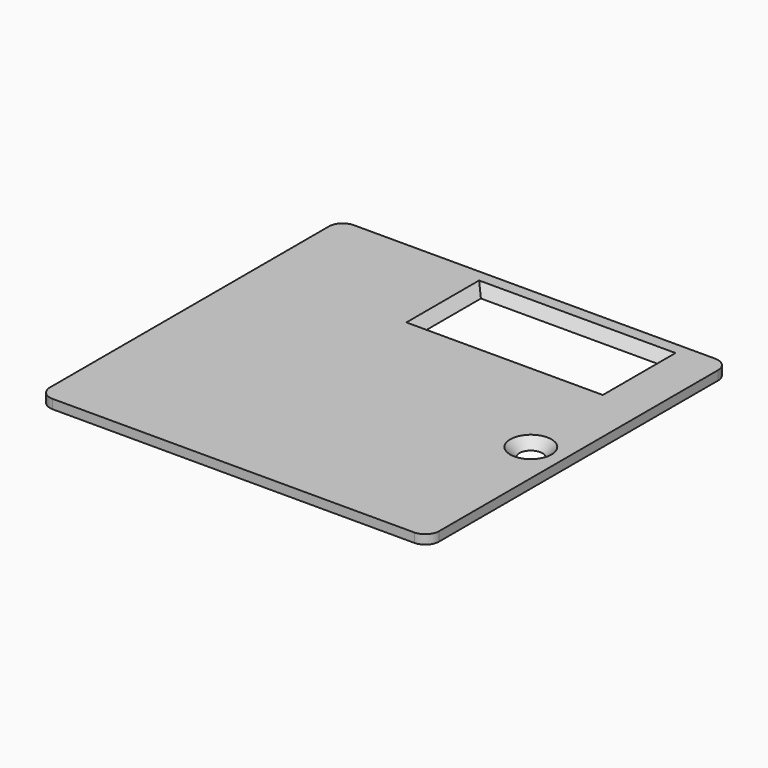
from build123d import *

# Parameters (mm, degrees)
F1_DEPTH     = 2
F2_R         = 3
F0_W         = 55
F0_H         = 20
F0_W_2       = 38
F0_H_2       = 15
F3_DEPTH     = 2
F4_R         = 3
F5_T1_DEPTH  = 38
F5_T3_DEPTH  = 15
F5_T9_DEPTH  = 44.1720391711
F5_T13_DEPTH = 21.1720391711
F5_T20_DEPTH = 44.1720391711
F5_T24_DEPTH = 21.1720391711
F5_T31_DEPTH = 21.1720391711
F5_T35_DEPTH = 44.1720391711
F5_T42_DEPTH = 44.1720391711
F5_T46_DEPTH = 21.1720391711
F8_START     = -23.1
F7_W         = 7.2
F7_H         = 3.4
F8_DEPTH     = 9.4
F9_START     = -23.1
F7_H_2       = 2.4
F9_DEPTH     = 11.8
F10_SIZE     = 2
F11_T4_DEPTH = 17.4867319519
F11_T9_DEPTH = 17.4867319519


# Not quite as in the source:
# - a fillet or chamfer that OpenCascade refuses, or shapes differently, is made with other operations: its cross-section is extruded or revolved along the edge and cut away or added
# - a feature names something its author has since deleted; it is built from what else it names


with BuildPart() as f1:
    # F0 (on Top) → F1 (new body)
    with BuildSketch(Plane.XY):
        with BuildLine():
            Line((42.8, 7.5), (46.1, 7.5))
            Line((46.1, 7.5), (46.1, 21.5))
            Line((46.1, 21.5), (-8.9, 21.5))
            Line((-8.9, 21.5), (-8.9, 41.5))
            Line((-8.9, 41.5), (-30.9, 41.5))
            Line((-30.9, 41.5), (-30.9, -33.5))
            Line((-30.9, -33.5), (46.1, -33.5))
            Line((46.1, -33.5), (46.1, -7.5))
            Line((46.1, -7.5), (42.8, -7.5))
            ThreePointArc((42.8, -7.5), (35.3, 0), (42.8, 7.5))
        make_face()
    extrude(amount=-F1_DEPTH)

    # F2
    f2_edges = [f1.edges().sort_by_distance(p)[0] for p in [
        (46.1, -33.5, -1),
        (-30.9, -33.5, -1),
        (-30.9, 41.5, -1),
    ]]
    fillet(f2_edges, radius=F2_R)

    # F0 (on Top) → F3 (join)
    with BuildSketch(Plane.XY):
        with Locations((18.6, 31.5)):
            Rectangle(F0_W, F0_H)
        with Locations((19, 32.5)):
            Rectangle(F0_W_2, F0_H_2, mode=Mode.SUBTRACT)
        with BuildLine():
            Line((42.8, 7.5), (46.1, 7.5))
            Line((46.1, 7.5), (46.1, 21.5))
            Line((46.1, 21.5), (-8.9, 21.5))
            Line((-8.9, 21.5), (-8.9, 41.5))
            Line((-8.9, 41.5), (-30.9, 41.5))
            Line((-30.9, 41.5), (-30.9, -33.5))
            Line((-30.9, -33.5), (46.1, -33.5))
            Line((46.1, -33.5), (46.1, -7.5))
            Line((46.1, -7.5), (42.8, -7.5))
            ThreePointArc((42.8, -7.5), (35.3, 0), (42.8, 7.5))
        make_face()
        with BuildLine():
            Line((42.8, 1.5), (42.8, 7.5))
            ThreePointArc((42.8, 7.5), (35.3, 0), (42.8, -7.5))
            Line((42.8, -7.5), (42.8, -1.5))
            ThreePointArc((42.8, -1.5), (41.3, 0), (42.8, 1.5))
        make_face()
        with BuildLine():
            Line((46.1, -6.7349832962), (46.1, 6.7349832962))
            ThreePointArc((46.1, 6.7349832962), (44.4937569599, 7.3062430401), (42.8, 7.5))
            Line((42.8, 7.5), (42.8, 1.5))
            ThreePointArc((42.8, 1.5), (43.8606601718, 1.0606601718), (44.3, 0))
            ThreePointArc((44.3, 0), (43.8606601718, -1.0606601718), (42.8, -1.5))
            Line((42.8, -1.5), (42.8, -7.5))
            ThreePointArc((42.8, -7.5), (44.4937569599, -7.3062430401), (46.1, -6.7349832962))
        make_face()
        with BuildLine():
            Line((46.1, -7.5), (46.1, -6.7349832962))
            ThreePointArc((46.1, -6.7349832962), (44.4937569599, -7.3062430401), (42.8, -7.5))
            Line((42.8, -7.5), (46.1, -7.5))
        make_face()
        with BuildLine():
            Line((50, 45), (-34.8, 45))
            Line((-34.8, 45), (-34.8, -37))
            Line((-34.8, -37), (50, -37))
            Line((50, -37), (50, -2.1))
            ThreePointArc((50, -2.1), (48.538751392, -4.8287402561), (46.1, -6.7349832962))
            Line((46.1, -6.7349832962), (46.1, -7.5))
            Line((46.1, -7.5), (46.1, -33.5))
            Line((46.1, -33.5), (-30.9, -33.5))
            Line((-30.9, -33.5), (-30.9, 41.5))
            Line((-30.9, 41.5), (-8.9, 41.5))
            Line((-8.9, 41.5), (46.1, 41.5))
            Line((46.1, 41.5), (46.1, 21.5))
            Line((46.1, 21.5), (46.1, 7.5))
            Line((46.1, 7.5), (46.1, 6.7349832962))
            ThreePointArc((46.1, 6.7349832962), (48.538751392, 4.8287402561), (50, 2.1))
            Line((50, 2.1), (50, 45))
        make_face()
        with BuildLine():
            Line((50, -2.1), (50, 2.1))
            ThreePointArc((50, 2.1), (48.538751392, 4.8287402561), (46.1, 6.7349832962))
            Line((46.1, 6.7349832962), (46.1, -6.7349832962))
            ThreePointArc((46.1, -6.7349832962), (48.538751392, -4.8287402561), (50, -2.1))
        make_face()
        with BuildLine():
            ThreePointArc((42.8, 7.5), (44.4937569599, 7.3062430401), (46.1, 6.7349832962))
            Line((46.1, 6.7349832962), (46.1, 7.5))
            Line((46.1, 7.5), (42.8, 7.5))
        make_face()
    extrude(amount=F3_DEPTH)

    # F4
    f4_edges = [f1.edges().sort_by_distance(p)[0] for p in [
        (50, -37, 1),
        (-34.8, -37, 1),
        (-34.8, 45, 1),
        (50, 45, 1),
    ]]
    fillet(f4_edges, radius=F4_R)

    # F5: chamfer of 2.4 on 4 edges, made by hand

    # F5_s2 → F5_t1 (cut)
    with BuildSketch(Plane.YZ):
        Polygon((42.4, 2), (40, -0.4), (40, 2), align=None)
        Polygon((22.6, 2), (25, -0.4), (25, 2), align=None)
    extrude(amount=F5_T1_DEPTH, mode=Mode.SUBTRACT)

    # F5_s4 → F5_t3 (cut)
    with BuildSketch(Plane.XZ.offset(-40)):
        Polygon((40.4, 2), (38, -0.4), (38, 2), align=None)
        Polygon((-2.4, 2), (0, -0.4), (0, 2), align=None)
    extrude(amount=F5_T3_DEPTH, mode=Mode.SUBTRACT)


with BuildPart() as f5_tool7:
    # F5_s8 → F5_t9 (new body)
    with BuildSketch(Plane.YZ.offset(-6.1720391711)):
        Polygon((42.4, 2), (40, -0.4), (40, 2), align=None)
    extrude(amount=F5_T9_DEPTH)

    split(bisect_by=Plane.YZ, keep=Keep.BOTTOM)


with BuildPart() as f5_tool11:
    # F5_s12 → F5_t13 (new body)
    with BuildSketch(Plane.XZ.offset(-25)):
        Polygon((-2.4, 2), (0, -0.4), (0, 2), align=None)
    extrude(amount=-F5_T13_DEPTH)

    split(bisect_by=Plane.XZ.offset(-40), keep=Keep.BOTTOM)


with BuildPart() as f5_tool7_1:
    add(f5_tool7.part)

    # F5_t15: intersect F5_tool11
    add(f5_tool11.part, mode=Mode.INTERSECT)


with BuildPart() as f1_1:
    add(f1.part)

    # F5_t5: cut F5_tool7
    add(f5_tool7_1.part, mode=Mode.SUBTRACT)


with BuildPart() as f5_tool18:
    # F5_s19 → F5_t20 (new body)
    with BuildSketch(Plane.YZ):
        Polygon((42.4, 2), (40, -0.4), (40, 2), align=None)
    extrude(amount=F5_T20_DEPTH)

    split(bisect_by=Plane.YZ.offset(38), keep=Keep.TOP)


with BuildPart() as f5_tool22:
    # F5_s23 → F5_t24 (new body)
    with BuildSketch(Plane.XZ.offset(-46.1720391711)):
        Polygon((40.4, 2), (38, -0.4), (38, 2), align=None)
    extrude(amount=F5_T24_DEPTH)

    split(bisect_by=Plane.XZ.offset(-40), keep=Keep.BOTTOM)


with BuildPart() as f5_tool18_1:
    add(f5_tool18.part)

    # F5_t26: intersect F5_tool22
    add(f5_tool22.part, mode=Mode.INTERSECT)


with BuildPart() as f1_2:
    add(f1_1.part)

    # F5_t16: cut F5_tool18
    add(f5_tool18_1.part, mode=Mode.SUBTRACT)


with BuildPart() as f5_tool29:
    # F5_s30 → F5_t31 (new body)
    with BuildSketch(Plane.XZ.offset(-40)):
        Polygon((40.4, 2), (38, -0.4), (38, 2), align=None)
    extrude(amount=F5_T31_DEPTH)

    split(bisect_by=Plane.XZ.offset(-25), keep=Keep.TOP)


with BuildPart() as f5_tool33:
    # F5_s34 → F5_t35 (new body)
    with BuildSketch(Plane.YZ.offset(44.1720391711)):
        Polygon((22.6, 2), (25, -0.4), (25, 2), align=None)
    extrude(amount=-F5_T35_DEPTH)

    split(bisect_by=Plane.YZ.offset(38), keep=Keep.TOP)


with BuildPart() as f5_tool29_1:
    add(f5_tool29.part)

    # F5_t37: intersect F5_tool33
    add(f5_tool33.part, mode=Mode.INTERSECT)


with BuildPart() as f1_3:
    add(f1_2.part)

    # F5_t27: cut F5_tool29
    add(f5_tool29_1.part, mode=Mode.SUBTRACT)


with BuildPart() as f5_tool40:
    # F5_s41 → F5_t42 (new body)
    with BuildSketch(Plane.YZ.offset(38)):
        Polygon((22.6, 2), (25, -0.4), (25, 2), align=None)
    extrude(amount=-F5_T42_DEPTH)

    split(bisect_by=Plane.YZ, keep=Keep.BOTTOM)


with BuildPart() as f5_tool44:
    # F5_s45 → F5_t46 (new body)
    with BuildSketch(Plane.XZ.offset(-18.8279608289)):
        Polygon((-2.4, 2), (0, -0.4), (0, 2), align=None)
    extrude(amount=-F5_T46_DEPTH)

    split(bisect_by=Plane.XZ.offset(-25), keep=Keep.TOP)


with BuildPart() as f5_tool40_1:
    add(f5_tool40.part)

    # F5_t48: intersect F5_tool44
    add(f5_tool44.part, mode=Mode.INTERSECT)


with BuildPart() as f1_4:
    add(f1_3.part)

    # F5_t38: cut F5_tool40
    add(f5_tool40_1.part, mode=Mode.SUBTRACT)

    # F6: chamfer of 3 on 1 edges, made by hand

    # F6_s1 → F6_t2 (revolve, cut)
    with BuildSketch(Plane.YZ.offset(42.8)):
        Polygon((4.5, 2), (1.5, -1), (1.5, 2), align=None)
    revolve(axis=Axis((42.8, 0, 2), (0, 0, -1)), mode=Mode.SUBTRACT)

    # F7 (on Right) → F8 (join)
    with BuildSketch(Plane.YZ.offset(F8_START)):
        with Locations((28.0882296383, -3.7)):
            Rectangle(F7_W, F7_H)
        with Locations((-20.1117703617, -3.7)):
            Rectangle(F7_W, F7_H)
    extrude(amount=-F8_DEPTH)

    # F7 (on Right) → F9 (join)
    with BuildSketch(Plane.YZ.offset(F9_START)):
        with Locations((28.0882296383, -6.6)):
            Rectangle(F7_W, F7_H_2)
        with Locations((-20.1117703617, -6.6)):
            Rectangle(F7_W, F7_H_2)
    extrude(amount=-F9_DEPTH)

    # F10
    f10_edges = [f1_4.edges().sort_by_distance(p)[0] for p in [
        (-23.1, -20.11177, -7.8),
        (-23.1, 28.08823, -7.8),
    ]]
    chamfer(f10_edges, length=F10_SIZE)

    # F11: chamfer of 2 on 2 edges, made by hand


with BuildPart() as f11_tool2:
    # F11_s3 → F11_t4 (new body)
    with BuildSketch(Plane.XZ.offset(11.3684043857)):
        Polygon((-30.5, -2), (-32.5, -4), (-32.5, -2), align=None)
    extrude(amount=F11_T4_DEPTH)

    split(bisect_by=Plane.YZ.offset(-30.9), keep=Keep.BOTTOM)


with BuildPart() as f1_5:
    add(f1_4.part)

    # F11_t1: cut F11_tool2
    add(f11_tool2.part, mode=Mode.SUBTRACT)


with BuildPart() as f11_tool7:
    # F11_s8 → F11_t9 (new body)
    with BuildSketch(Plane.XZ.offset(-36.8315956143)):
        Polygon((-30.5, -2), (-32.5, -4), (-32.5, -2), align=None)
    extrude(amount=F11_T9_DEPTH)

    split(bisect_by=Plane.YZ.offset(-30.9), keep=Keep.BOTTOM)


with BuildPart() as f1_6:
    add(f1_5.part)

    # F11_t6: cut F11_tool7
    add(f11_tool7.part, mode=Mode.SUBTRACT)


solid = f1_6.part
